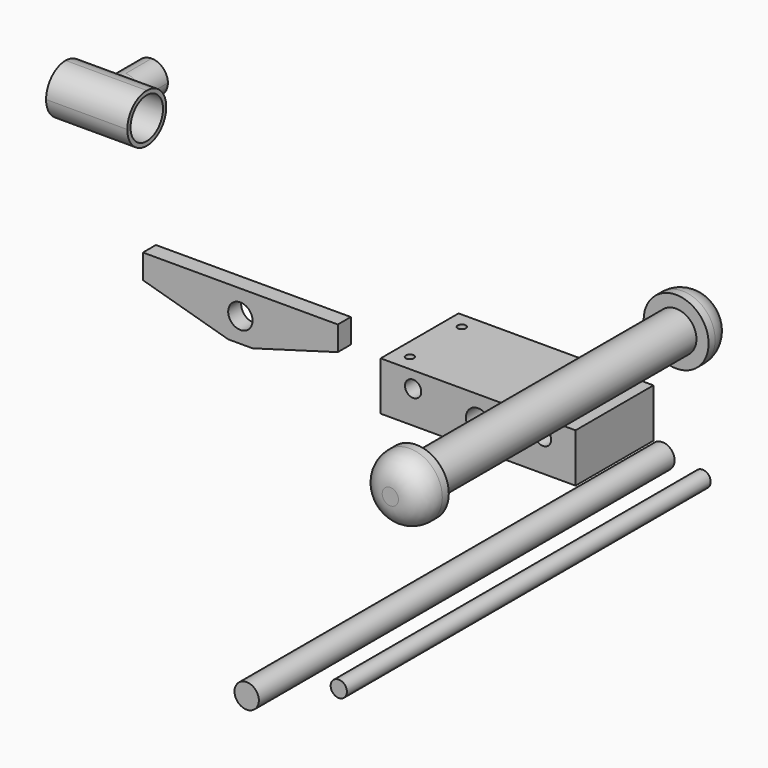
from build123d import *

# Parameters (mm, degrees)
F0_W          = 152.4
F0_H          = 76.2
F1_DEPTH      = 38.1
F2_R          = 6.35
F2_R_2        = 9.525
F3_DEPTH      = 76.2
F4_R          = 3.175
F5_DEPTH      = 38.1
F6_R          = 6.35
F7_DEPTH      = 355.6
F8_R          = 9.525
F9_DEPTH      = 406.4
F11_DEPTH     = 12.7
F12_R         = 6.35
F13_DEPTH     = 6.35
F14_R         = 9.525
F15_DEPTH     = 25.4
F16_W         = 25.4
F16_H         = 25.4
F17_DEPTH     = 25.4
F19_W         = 63.5
F19_H         = 38.1
F20_DEPTH     = 19.05
F21_R         = 12.69999
F22_T1_DEPTH  = 158.75
F22_T6_DEPTH  = 158.75
F22_S7_R      = 12.69999
F22_T8_DEPTH  = 82
F22_T12_DEPTH = 158.75
F22_S13_R     = 12.69999
F22_T14_DEPTH = 82
F23_R         = 15.875
F24_DEPTH     = 63.5
F25_R         = 9.525
F26_DEPTH     = 25.4
F27_R         = 15.875
F28_DEPTH     = 254
F29_R         = 25.4
F30_DEPTH     = 25.4
F31_R         = 25.4
F32_DEPTH     = 25.4
F33_R         = 19.05


# Not quite as in the source:
# - a fillet or chamfer that OpenCascade refuses, or shapes differently, is made with other operations: its cross-section is extruded or revolved along the edge and cut away or added
# - a fillet or chamfer is up to 0.001 mm smaller than in the source, because OpenCascade refuses the exact size


with BuildPart() as f1:
    # F0 (on Top) → F1 (new body)
    with BuildSketch(Plane.XY):
        with Locations((17.3710167248, -3.5089952871)):
            Rectangle(F0_W, F0_H)
    extrude(amount=F1_DEPTH)

    # F2 (on face) → F3 (cut, through all)
    with BuildSketch(Plane.XZ.offset(41.6089952871)):
        with Locations((-33.4289832752, 25.4)):
            Circle(F2_R)
        with Locations((68.1710167248, 25.4)):
            Circle(F2_R)
        with Locations((17.3710167248, 19.05)):
            Circle(F2_R_2)
    extrude(amount=-F3_DEPTH, mode=Mode.SUBTRACT)

    # F4 (on face) → F5 (cut, through all)
    with BuildSketch(Plane.XY.offset(38.1)):
        with Locations((-46.1289832752, 21.8910047129)):
            Circle(F4_R)
        with Locations((-46.1289832752, -28.9089952871)):
            Circle(F4_R)
        with Locations((80.8710167248, 21.8910047129)):
            Circle(F4_R)
        with Locations((80.8710167248, -28.9089952871)):
            Circle(F4_R)
    extrude(amount=-F5_DEPTH, mode=Mode.SUBTRACT)


with BuildPart() as f7:
    # F6 (on Front) → F7 (new body)
    with BuildSketch(Plane.XZ):
        with Locations((159.6328914165, 9.2687001452)):
            Circle(F6_R)
    extrude(amount=F7_DEPTH)


with BuildPart() as f9:
    # F8 (on Front) → F9 (new body)
    with BuildSketch(Plane.XZ):
        with Locations((128.2307356596, 14.8274637759)):
            Circle(F8_R)
    extrude(amount=F9_DEPTH)


with BuildPart() as f11:
    # F10 (on Front) → F11 (new body)
    with BuildSketch(Plane.XZ):
        Polygon((-115.4667288065, 12.1940965524), (-115.4667288065, 31.2440965524), (-267.8667288065, 31.2440965524), (-267.8667288065, 12.1940965524), (-201.1917288065, -6.8559034476), (-182.1417288065, -6.8559034476), align=None)
    extrude(amount=F11_DEPTH)

    # F12 (on face) → F13 (cut)
    with BuildSketch(Plane(origin=(0, 0, 0), x_dir=(-1, 0, 0), z_dir=(0, 1, 0))):
        with Locations((242.4667288065, 18.5440965524)):
            Circle(F12_R)
        with Locations((140.8667288065, 18.5440965524)):
            Circle(F12_R)
    extrude(amount=-F13_DEPTH, mode=Mode.SUBTRACT)

    # F14 (on face) → F15 (cut)
    with BuildSketch(Plane(origin=(0, 0, 0), x_dir=(-1, 0, 0), z_dir=(0, 1, 0))):
        with Locations((191.6667288065, 12.1940965524)):
            Circle(F14_R)
    extrude(amount=-F15_DEPTH, mode=Mode.SUBTRACT)


with BuildPart() as f17:
    # F16 (on Front) → F17 (new body)
    with BuildSketch(Plane.XZ):
        with Locations((-271.2143993781, 145.8536982536)):
            Rectangle(F16_W, F16_H)
    extrude(amount=F17_DEPTH)

    # F19 (on offset) → F20 (join, symmetric)
    with BuildSketch(Plane.XY.offset(145.8536982536)):
        with Locations((-271.2143993781, -44.45)):
            Rectangle(F19_W, F19_H)
    extrude(amount=F20_DEPTH, both=True)

    # F21 (radius 12.7 in the source; OpenCascade refuses exactly that, so slightly less here)
    f21_edges = [f17.edges().sort_by_distance(p)[0] for p in [
        (-283.914399, -12.7, 158.553698),
        (-258.514399, -12.7, 158.553698),
        (-283.914399, -12.7, 133.153698),
        (-258.514399, -12.7, 133.153698),
    ]]
    fillet(f21_edges, radius=F21_R)

    # F22: fillet of radius 19.05 on 4 edges, made by hand

    # F22_s2 → F22_t1 (cut)
    with BuildSketch(Plane.YZ.offset(-350.5893993781)):
        with BuildLine():
            ThreePointArc((-44.45, 164.9036982536), (-57.9203841816, 159.3240824352), (-63.5, 145.8536982536))
            Line((-63.5, 145.8536982536), (-63.5, 164.9036982536))
            Line((-63.5, 164.9036982536), (-44.45, 164.9036982536))
        make_face()
        with BuildLine():
            ThreePointArc((-44.45, 126.8036982536), (-57.9203841816, 132.383314072), (-63.5, 145.8536982536))
            Line((-63.5, 145.8536982536), (-63.5, 126.8036982536))
            Line((-63.5, 126.8036982536), (-44.45, 126.8036982536))
        make_face()
    extrude(amount=F22_T1_DEPTH, mode=Mode.SUBTRACT)


with BuildPart() as f22_tool4:
    # F22_s5 → F22_t6 (new body)
    with BuildSketch(Plane.YZ.offset(-191.8393993781)):
        with BuildLine():
            ThreePointArc((-25.4, 145.8536982536), (-30.9796158184, 159.3240824352), (-44.45, 164.9036982536))
            Line((-44.45, 164.9036982536), (-25.4, 164.9036982536))
            Line((-25.4, 164.9036982536), (-25.4, 145.8536982536))
        make_face()
    extrude(amount=-F22_T6_DEPTH)

    # F22_s7 → F22_t8 (cut, symmetric)
    with BuildSketch(Plane.XZ.offset(34.9)):
        with Locations((-271.2144093781, 145.8537082536)):
            Circle(F22_S7_R)
    extrude(amount=F22_T8_DEPTH, both=True, mode=Mode.SUBTRACT)


with BuildPart() as f17_1:
    add(f17.part)

    # F22_t3: cut F22_tool4
    add(f22_tool4.part, mode=Mode.SUBTRACT)


with BuildPart() as f22_tool10:
    # F22_s11 → F22_t12 (new body)
    with BuildSketch(Plane.YZ.offset(-191.8393993781)):
        with BuildLine():
            ThreePointArc((-25.4, 145.8536982536), (-30.9796158184, 132.383314072), (-44.45, 126.8036982536))
            Line((-44.45, 126.8036982536), (-25.4, 126.8036982536))
            Line((-25.4, 126.8036982536), (-25.4, 145.8536982536))
        make_face()
    extrude(amount=-F22_T12_DEPTH)

    # F22_s13 → F22_t14 (cut, symmetric)
    with BuildSketch(Plane.XZ.offset(34.9)):
        with Locations((-271.2144093781, 145.8536882536)):
            Circle(F22_S13_R)
    extrude(amount=F22_T14_DEPTH, both=True, mode=Mode.SUBTRACT)


with BuildPart() as f17_2:
    add(f17_1.part)

    # F22_t9: cut F22_tool10
    add(f22_tool10.part, mode=Mode.SUBTRACT)

    # F23 (on face) → F24 (cut, through all)
    with BuildSketch(Plane(origin=(-302.9643993781, 0, 0), x_dir=(0, -1, 0), z_dir=(-1, 0, 0))):
        with Locations((44.45, 145.8536982536)):
            Circle(F23_R)
    extrude(amount=-F24_DEPTH, mode=Mode.SUBTRACT)

    # F25 (on face) → F26 (cut)
    with BuildSketch(Plane(origin=(0, 0, 0), x_dir=(-1, 0, 0), z_dir=(0, 1, 0))):
        with Locations((271.2143993781, 145.8536982536)):
            Circle(F25_R)
    extrude(amount=-F26_DEPTH, mode=Mode.SUBTRACT)


with BuildPart() as f28:
    # F27 (on Front) → F28 (new body)
    with BuildSketch(Plane.XZ):
        with Locations((138.9757394791, 103.8877665997)):
            Circle(F27_R)
    extrude(amount=F28_DEPTH)

    # F29 (on face) → F30 (join)
    with BuildSketch(Plane.XZ.offset(254)):
        with Locations((138.9757394791, 103.8877665997)):
            Circle(F29_R)
    extrude(amount=F30_DEPTH)

    # F31 (on face) → F32 (join)
    with BuildSketch(Plane(origin=(0, 0, 0), x_dir=(-1, 0, 0), z_dir=(0, 1, 0))):
        with Locations((-138.9757394791, 103.8877665997)):
            Circle(F31_R)
    extrude(amount=F32_DEPTH)

    # F33
    f33_edges = [f28.edges().sort_by_distance(p)[0] for p in [
        (113.575739, -279.4, 103.887767),
        (164.375739, 25.4, 103.887767),
    ]]
    fillet(f33_edges, radius=F33_R)


solid = Compound([f1.part, f7.part, f9.part, f11.part, f17_2.part, f28.part])
